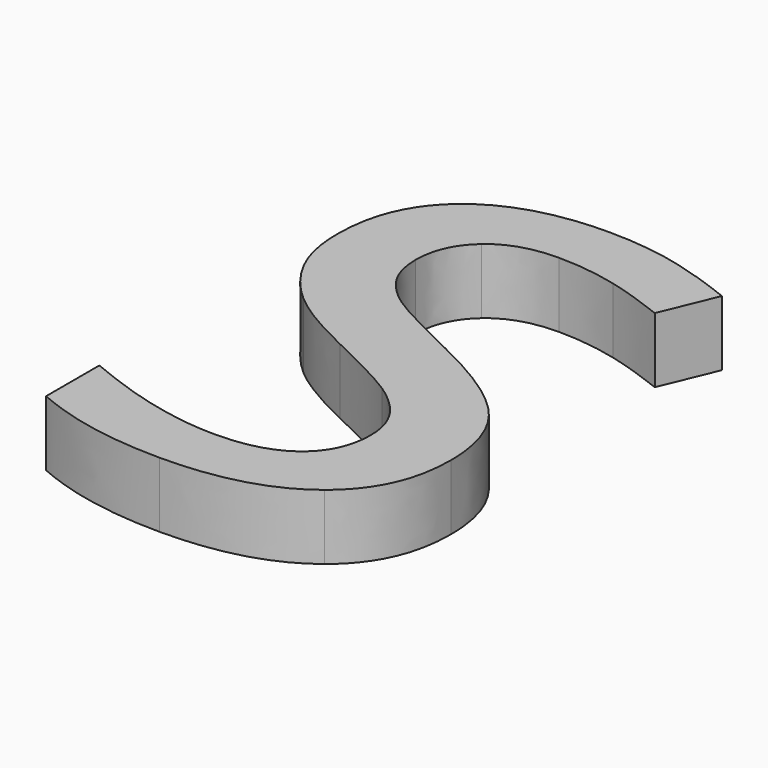
from build123d import *

# Parameters (mm, degrees)
F1_DEPTH = 2


# Not quite as in the source:
# - ends of sketch curves that miss each other by under 0.0002 mm in the source are joined
# - the dataset's text gives a spline's control points without its knots; the knots are read off the source's solid


with BuildPart() as f1:
    # F0 (on Top) → F1 (new body)
    with BuildSketch(Plane.XY):
        with BuildLine():
            add(Edge.make_bspline(
                [(-4.5539323159, 3.4404925622), (-4.553932314, 4.109133441), (-4.4417509068, 4.6815041688), (-4.121937897, 5.4234547922), (-3.9898413305, 5.6517314099), (-3.6715155244, 6.0768112467), (-3.4851703783, 6.273694276), (-3.2685167558, 6.4563475141)],
                knots=[0, 0, 0, 0, 0.5, 0.5, 0.75, 0.75, 1, 1, 1, 1], degree=3))
            add(Edge.make_bspline(
                [(-4.1653522884, 1.6684308192), (-4.4188295054, 2.1571348906), (-4.5539323132, 2.7395984093), (-4.5539323159, 3.4404925622)],
                knots=[0, 0, 0, 0, 1, 1, 1, 1], degree=3))
            add(Edge.make_bspline(
                [(-3.0880831784, 0.3100080442), (-3.5410735232, 0.7013744056), (-3.8969951229, 1.1510382057), (-4.1653522884, 1.6684308192)],
                knots=[0, 0, 0, 0, 1, 1, 1, 1], degree=3))
            add(Edge.make_bspline(
                [(-0.94726724, -0.9733503247), (-0.9476283907, -0.9731801173), (-0.9479895414, -0.9730099099), (-0.948350692, -0.9728397025), (-1.4381555261, -0.7419986681), (-1.8627330629, -0.5176434714), (-2.5774559291, -0.0871012519), (-2.8674308006, 0.1193728081), (-3.0880831784, 0.3100080442)],
                knots=[-0.0003686679, -0.0003686679, -0.0003686679, -0.0003686679, 0, 0, 0, 0.5, 0.5, 1, 1, 1, 1], degree=3))
            add(Edge.make_bspline(
                [(1.2638188496, -2.1313058458), (1.0591492674, -1.9955628295), (0.7810896534, -1.8386696922), (0.0493295513, -1.4564253852), (-0.4034193402, -1.2324993239), (-0.9461859739, -0.9738655589), (-0.9465463959, -0.9736938141), (-0.946906818, -0.9735220694), (-0.94726724, -0.9733503247)],
                knots=[0, 0, 0, 0, 0.5, 0.5, 1, 1, 1, 1.000332023, 1.000332023, 1.000332023, 1.000332023], degree=3))
            add(Edge.make_bspline(
                [(2.2073726786, -3.0012041242), (1.9740381312, -2.6745358034), (1.654810322, -2.3906232081), (1.2638188496, -2.1313058458)],
                knots=[0, 0, 0, 0, 1, 1, 1, 1], degree=3))
            add(Edge.make_bspline(
                [(2.5831118874, -4.1916276187), (2.5831119009, -3.9779409831), (2.5527095247, -3.7664931745), (2.4264212856, -3.3640546657), (2.3305505576, -3.173653134), (2.2073726786, -3.0012041242)],
                knots=[0, 0, 0, 0, 0.5, 0.5, 1, 1, 1, 1], degree=3))
            add(Edge.make_bspline(
                [(1.7310564521, -5.9594051259), (1.8694470021, -5.8607866548), (1.9951638757, -5.7464648732), (2.2124688094, -5.4892251058), (2.3038523063, -5.3464167266), (2.519150799, -4.8886706939), (2.5831119027, -4.5468724456), (2.5831118874, -4.1916276187)],
                knots=[0, 0, 0, 0, 0.25, 0.25, 0.5, 0.5, 1, 1, 1, 1], degree=3))
            add(Edge.make_bspline(
                [(-0.3604753147, -6.502818499), (0.0582122658, -6.5028185014), (0.4414416098, -6.4634017893), (1.1407820285, -6.2894614297), (1.4577253675, -6.1541835635), (1.7310564521, -5.9594051259)],
                knots=[0, 0, 0, 0, 0.5, 0.5, 1, 1, 1, 1], degree=3))
            add(Edge.make_bspline(
                [(-2.6224302874, -6.1809013634), (-1.8135993387, -6.3928882585), (-1.0605109021, -6.5028184969), (-0.3604753147, -6.502818499)],
                knots=[0, 0, 0, 0, 1, 1, 1, 1], degree=3))
            add(Edge.make_bspline(
                [(-4.7454580591, -5.4407007971), (-3.9473161615, -5.7716151358), (-3.2419123285, -6.018541014), (-2.6224302874, -6.1809013634)],
                knots=[0.2417760748, 0.2417760748, 0.2417760748, 0.2417760748, 1, 1, 1, 1], degree=3))
            Line((-4.7454580591, -5.4407007971), (-4.7454580591, -7.4795386684))
            add(Edge.make_bspline(
                [(-0.6315023097, -8.2730601286), (-2.1864345754, -8.2730601282), (-3.5521940185, -8.0048830709), (-4.7454580591, -7.4795386684)],
                knots=[0, 0, 0, 0, 0.9183123613, 0.9183123613, 0.9183123613, 0.9183123613], degree=3))
            add(Edge.make_bspline(
                [(3.4928160756, -7.1080140655), (3.0203241877, -7.4861136355), (2.4493404192, -7.7758563937), (1.0800859896, -8.1699938198), (0.2819186052, -8.2730601281), (-0.6315023097, -8.2730601286)],
                knots=[0, 0, 0, 0, 0.5, 0.5, 1, 1, 1, 1], degree=3))
            add(Edge.make_bspline(
                [(4.8917938139, -4.0217840352), (4.8917938118, -4.7009415685), (4.7711067522, -5.2821953174), (4.4246282935, -6.0408703732), (4.2811707681, -6.2753258521), (3.9340237801, -6.7139024983), (3.7301988047, -6.918054596), (3.4928160756, -7.1080140655)],
                knots=[0, 0, 0, 0, 0.5, 0.5, 0.75, 0.75, 1, 1, 1, 1], degree=3))
            add(Edge.make_bspline(
                [(4.1507940458, -1.638882878), (4.396515413, -1.9570273867), (4.5792206673, -2.30751695), (4.827118095, -3.0950479417), (4.8917938123, -3.5328168935), (4.8917938139, -4.0217840352)],
                knots=[0, 0, 0, 0, 0.5, 0.5, 1, 1, 1, 1], degree=3))
            add(Edge.make_bspline(
                [(1.1782471579, 0.4183491959), (1.9294970419, 0.0585462091), (2.5547792836, -0.2982557111), (3.5466215561, -0.992037242), (3.9119064629, -1.3295863067), (4.1507940458, -1.638882878)],
                knots=[0, 0, 0, 0, 0.5, 0.5, 1, 1, 1, 1], degree=3))
            add(Edge.make_bspline(
                [(-1.1143311666, 1.6184455474), (-1.0162509018, 1.5510390918), (-0.9004048855, 1.4804604262), (-0.6206808382, 1.3208013117), (-0.45698794, 1.2321520315), (0.1108160421, 0.9359869549), (0.5914968065, 0.6983949543), (1.1782471579, 0.4183491959)],
                knots=[0, 0, 0, 0, 0.25, 0.25, 0.5, 0.5, 0.9998046197, 0.9998046197, 0.9998046197, 0.9998046197], degree=3))
            add(Edge.make_bspline(
                [(-1.9560474883, 2.451198266), (-1.8566181148, 2.2916099906), (-1.7343676506, 2.1446246375), (-1.4523338231, 1.8693058849), (-1.2924097348, 1.7408315854), (-1.1143311666, 1.6184455474)],
                knots=[0, 0, 0, 0, 0.5, 0.5, 1, 1, 1, 1], degree=3))
            add(Edge.make_bspline(
                [(-2.2560914692, 3.5561307467), (-2.2560914812, 3.358554546), (-2.232979569, 3.1644905564), (-2.1338539681, 2.7921448588), (-2.0575762287, 2.6141561535), (-1.9560474883, 2.451198266)],
                knots=[0, 0, 0, 0, 0.5, 0.5, 1, 1, 1, 1], degree=3))
            add(Edge.make_bspline(
                [(-1.5318803699, 5.1870673998), (-1.6485374043, 5.0854884976), (-1.7539534558, 4.9731201094), (-1.9368474168, 4.7284320339), (-2.0142254381, 4.5961241937), (-2.1985253422, 4.1773747627), (-2.2560914855, 3.8703955411), (-2.2560914692, 3.5561307467)],
                knots=[0, 0, 0, 0, 0.25, 0.25, 0.5, 0.5, 1, 1, 1, 1], degree=3))
            add(Edge.make_bspline(
                [(0.3622633388, 5.7878203751), (-0.012208003, 5.7878203799), (-0.3599577221, 5.7447623809), (-0.9981166165, 5.5511975822), (-1.2885907071, 5.398911453), (-1.5318803699, 5.1870673998)],
                knots=[0, 0, 0, 0, 0.5, 0.5, 1, 1, 1, 1], degree=3))
            add(Edge.make_bspline(
                [(2.1965066912, 5.556154833), (1.5795493196, 5.7097488235), (0.967120358, 5.7878203748), (0.3622633388, 5.7878203751)],
                knots=[0, 0, 0, 0, 1, 1, 1, 1], degree=3))
            add(Edge.make_bspline(
                [(3.9397827582, 4.9814492737), (3.2685520169, 5.2415958191), (2.6904101659, 5.4331955967), (2.1965066912, 5.556154833)],
                knots=[0.1998130955, 0.1998130955, 0.1998130955, 0.1998130955, 1, 1, 1, 1], degree=3))
            Line((3.9397827582, 4.9814492737), (4.6406248453, 6.6751509842))
            add(Edge.make_bspline(
                [(2.7885063884, 7.2906242127), (3.380503744, 7.1369061979), (3.9980767952, 6.9320131673), (4.6406248453, 6.6751509842)],
                knots=[0, 0, 0, 0, 0.7923628244, 0.7923628244, 0.7923628244, 0.7923628244], degree=3))
            add(Edge.make_bspline(
                [(0.4742878301, 7.5761304711), (1.2877472267, 7.5761304708), (2.0577984223, 7.4803598207), (2.7885063884, 7.2906242127)],
                knots=[0, 0, 0, 0, 1, 1, 1, 1], degree=3))
            add(Edge.make_bspline(
                [(-3.2685167558, 6.4563475141), (-2.836280375, 6.8207511786), (-2.3183058122, 7.0983331165), (-1.0776039847, 7.4767690155), (-0.3546345611, 7.5761304704), (0.4742878301, 7.5761304711)],
                knots=[0, 0, 0, 0, 0.5, 0.5, 1, 1, 1, 1], degree=3))
        make_face()
    extrude(amount=F1_DEPTH)


solid = f1.part
